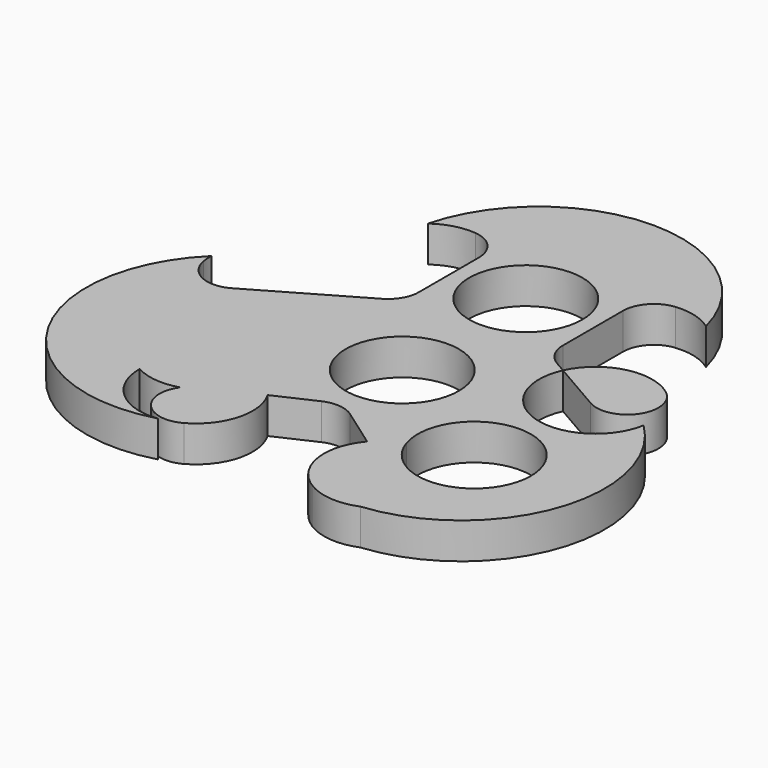
from build123d import *

# Parameters (mm, degrees)
F0_R     = 11
F1_DEPTH = 7


# Not quite as in the source:
# - a feature of the source that left no trace in its solid (it failed there, or was rolled back) is left out


with BuildPart() as f1:
    # F0 (on Top) → F1 (new body)
    with BuildSketch(Plane.XY):
        with BuildLine():
            ThreePointArc((-14.9810198925, -15.0753065176), (-14.9808265585, -15.0376534794), (-14.9807621135, -15))
            ThreePointArc((-14.9807621135, -15), (-31.5612257999, -5.5206316115), (-31.3186575763, -24.6180492839))
            ThreePointArc((-31.3186575763, -24.6180492839), (-25.8668980567, -15.1949407788), (-14.9810198925, -15.0753065176))
        make_face()
        with BuildLine():
            ThreePointArc((-31.3186575763, -24.6180492839), (-31.5612257999, -5.5206316115), (-14.9807621135, -15))
            ThreePointArc((-14.9807621135, -15), (-14.9808265585, -15.0376534794), (-14.9810198925, -15.0753065176))
            ThreePointArc((-14.9810198925, -15.0753065176), (-12.6066127008, -16.8498624622), (-10.7922626222, -19.1940024121))
            Line((-10.7922626222, -19.1940024121), (-3.1471315948, -15.6774235403))
            ThreePointArc((-3.1471315948, -15.6774235403), (-0.0857175759, -15.1540545193), (2.8272292465, -16.231510661))
            Line((2.8272292465, -16.231510661), (10.5215510319, -21.6791304199))
            ThreePointArc((10.5215510319, -21.6791304199), (12.7842474134, -19.6747261792), (15.5070984162, -18.3618995755))
            ThreePointArc((15.5070984162, -18.3618995755), (24.2793363394, -4.1323806501), (36.9807621135, -15))
            ThreePointArc((36.9807621135, -15), (34.8711182406, -21.4777749215), (29.3513861257, -25.470859266))
            ThreePointArc((29.3513861257, -25.470859266), (28.8526132199, -33.4697356256), (23.0588387456, -39.0071515183))
            ThreePointArc((23.0588387456, -39.0071515183), (46.7268088994, -20.5659720475), (39.9540974013, 8.6638122562))
            ThreePointArc((39.9540974013, 8.6638122562), (25.8569369314, 0.0414243654), (19.1161667268, 15.1290856588))
            Line((19.1161667268, 15.1290856588), (17, 16.3508550882))
            ThreePointArc((17, 16.3508550882), (14.8038475773, 18.5470075109), (14, 21.5470075109))
            Line((14, 21.5470075109), (14, 36.1008175109))
            ThreePointArc((14, 36.1008175109), (15.5502809077, 40.1257398704), (19.4, 42.0707421335))
            ThreePointArc((19.4, 42.0707421335), (23.3917111277, 41.73898575), (27, 40))
            ThreePointArc((27, 40), (0, 60.9456692242), (-27, 40))
            ThreePointArc((-27, 40), (-23.3917111277, 41.73898575), (-19.4, 42.0707421335))
            ThreePointArc((-19.4, 42.0707421335), (-15.5502809077, 40.1257398704), (-14, 36.1008175109))
            Line((-14, 36.1008175109), (-14, 21.5470075109))
            ThreePointArc((-14, 21.5470075109), (-14.8038475773, 18.5470075109), (-17, 16.3508550882))
            Line((-17, 16.3508550882), (-36.9299341095, 4.8443022651))
            ThreePointArc((-36.9299341095, 4.8443022651), (-42.4725061765, 4.6058132751), (-45.8413922703, 9.0134871064))
            ThreePointArc((-45.8413922703, 9.0134871064), (-45.9732793063, 10.0784919978), (-46.000762454, 11.1512800876))
            ThreePointArc((-46.000762454, 11.1512800876), (-50.6402441015, -22.7042404267), (-19.000762454, -35.6140917168))
            ThreePointArc((-19.000762454, -35.6140917168), (-27.6443184319, -32.8993578589), (-31.3186575763, -24.6180492839))
        make_face()
        Circle(F0_R, mode=Mode.SUBTRACT)
        with Locations((0, 30)):
            Circle(F0_R, mode=Mode.SUBTRACT)
        with BuildLine():
            ThreePointArc((-14.9810198925, -15.0753065176), (-25.8668980567, -15.1949407788), (-31.3186575763, -24.6180492839))
            ThreePointArc((-31.3186575763, -24.6180492839), (-27.1082014874, -25.9420692951), (-22.7162279438, -25.5044189109))
            ThreePointArc((-22.7162279438, -25.5044189109), (-21.6737707093, -24.4089875601), (-20.3905407876, -23.6089826237))
            Line((-20.3905407876, -23.6089826237), (-17.9001022816, -22.4634400032))
            ThreePointArc((-17.9001022816, -22.4634400032), (-15.7503386264, -19.0420830366), (-14.9810198925, -15.0753065176))
        make_face()
        with BuildLine():
            ThreePointArc((-10.7922626222, -19.1940024121), (-12.6066127008, -16.8498624622), (-14.9810198925, -15.0753065176))
            ThreePointArc((-14.9810198925, -15.0753065176), (-15.7503386264, -19.0420830366), (-17.9001022816, -22.4634400032))
            Line((-17.9001022816, -22.4634400032), (-10.7922626222, -19.1940024121))
        make_face()
        with BuildLine():
            ThreePointArc((-20.3905407876, -23.6089826237), (-21.6737707093, -24.4089875601), (-22.7162279438, -25.5044189109))
            ThreePointArc((-22.7162279438, -25.5044189109), (-20.1079225182, -24.3010620408), (-17.9001022816, -22.4634400032))
            Line((-17.9001022816, -22.4634400032), (-20.3905407876, -23.6089826237))
        make_face()
        with BuildLine():
            ThreePointArc((-17.9001022816, -22.4634400032), (-20.1079225182, -24.3010620408), (-22.7162279438, -25.5044189109))
            ThreePointArc((-22.7162279438, -25.5044189109), (-22.3834789255, -33.0283008678), (-14.9603721303, -34.299916815))
            ThreePointArc((-14.9603721303, -34.299916815), (-9.7151694528, -27.619201463), (-10.7922626222, -19.1940024121))
            Line((-10.7922626222, -19.1940024121), (-17.9001022816, -22.4634400032))
        make_face()
        with BuildLine():
            ThreePointArc((15.5070984162, -18.3618995755), (12.7842474134, -19.6747261792), (10.5215510319, -21.6791304199))
            Line((10.5215510319, -21.6791304199), (19.2043932568, -27.8266277806))
            ThreePointArc((19.2043932568, -27.8266277806), (21.4514676336, -34.5535505425), (15.7145306517, -38.7234890511))
            ThreePointArc((15.7145306517, -38.7234890511), (19.3772945803, -39.1084399418), (23.0588387456, -39.0071515183))
            ThreePointArc((23.0588387456, -39.0071515183), (28.8526132199, -33.4697356256), (29.3513861257, -25.470859266))
            ThreePointArc((29.3513861257, -25.470859266), (20.9560611112, -24.7853144986), (15.5070984162, -18.3618995755))
        make_face()
        with BuildLine():
            Line((19.2043932568, -27.8266277806), (10.5215510319, -21.6791304199))
            ThreePointArc((10.5215510319, -21.6791304199), (7.9240920964, -29.8417100549), (11.968923576, -37.3924608467))
            ThreePointArc((11.968923576, -37.3924608467), (12.5815553416, -37.8265611192), (13.2436070612, -38.1807478602))
            ThreePointArc((13.2436070612, -38.1807478602), (14.4729085443, -38.4801643471), (15.7145306517, -38.7234890511))
            ThreePointArc((15.7145306517, -38.7234890511), (21.4514676336, -34.5535505425), (19.2043932568, -27.8266277806))
        make_face()
        with BuildLine():
            ThreePointArc((13.2436070612, -38.1807478602), (14.450138713, -38.5838279613), (15.7145306517, -38.7234890511))
            ThreePointArc((15.7145306517, -38.7234890511), (14.4729085443, -38.4801643471), (13.2436070612, -38.1807478602))
        make_face()
        with BuildLine():
            ThreePointArc((23.0588387456, -39.0071515183), (19.3772945803, -39.1084399418), (15.7145306517, -38.7234890511))
            ThreePointArc((15.7145306517, -38.7234890511), (14.450138713, -38.5838279613), (13.2436070612, -38.1807478602))
            ThreePointArc((13.2436070612, -38.1807478602), (13.0987456479, -38.1415433693), (12.9540974013, -38.1015595481))
            ThreePointArc((12.9540974013, -38.1015595481), (17.8958322334, -39.7888480911), (23.0588387456, -39.0071515183))
        make_face()
    extrude(amount=F1_DEPTH)


with BuildPart() as f1b:
    # F0 (on Top) → F1, piece 2 (new body)
    with BuildSketch(Plane.XY):
        with BuildLine():
            ThreePointArc((35.6622980234, 19.3878045659), (26.3746934117, 21.2001691989), (19.1161667268, 15.1290856588))
            Line((19.1161667268, 15.1290856588), (29.0918954701, 9.3695959835))
            ThreePointArc((29.0918954701, 9.3695959835), (37.1091123847, 11.2752264975), (35.6622980234, 19.3878045659))
        make_face()
    extrude(amount=F1_DEPTH)


solid = Compound([f1.part, f1b.part])
